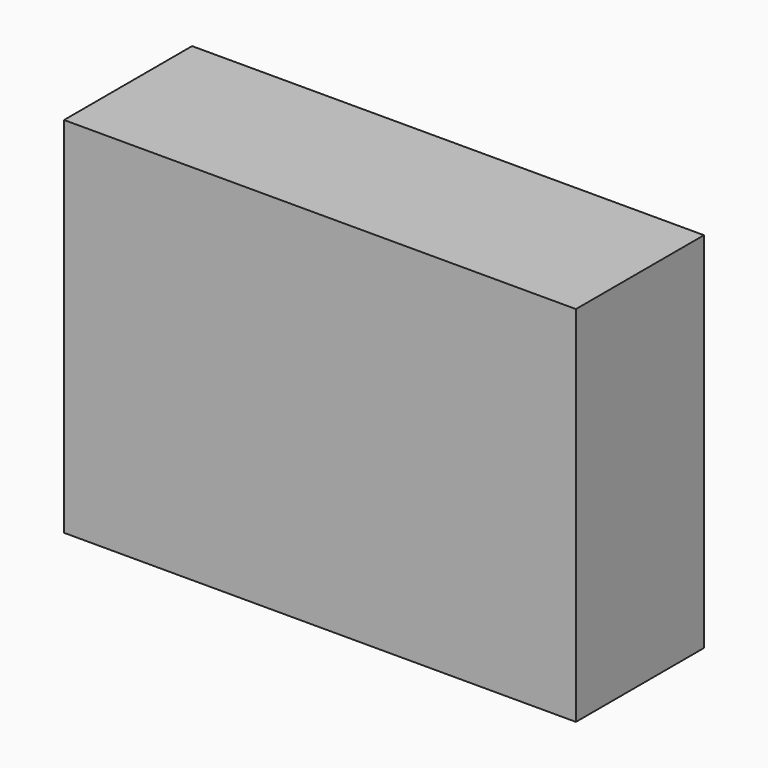
from build123d import *

# Parameters (mm, degrees)
F2_W     = 81.2448132783
F2_H     = 57.6836876571
F3_DEPTH = 25.4


# Not quite as in the source:
# - the program builds the solid bodies; features that only make, move or delete a surface that nothing else refers to are left out


with BuildPart() as f3:
    # F2 (on Front) → F3 (new body)
    with BuildSketch(Plane.XZ):
        with Locations((-56.3210612163, -9.1266985983)):
            Rectangle(F2_W, F2_H)
    extrude(amount=F3_DEPTH)


solid = f3.part
